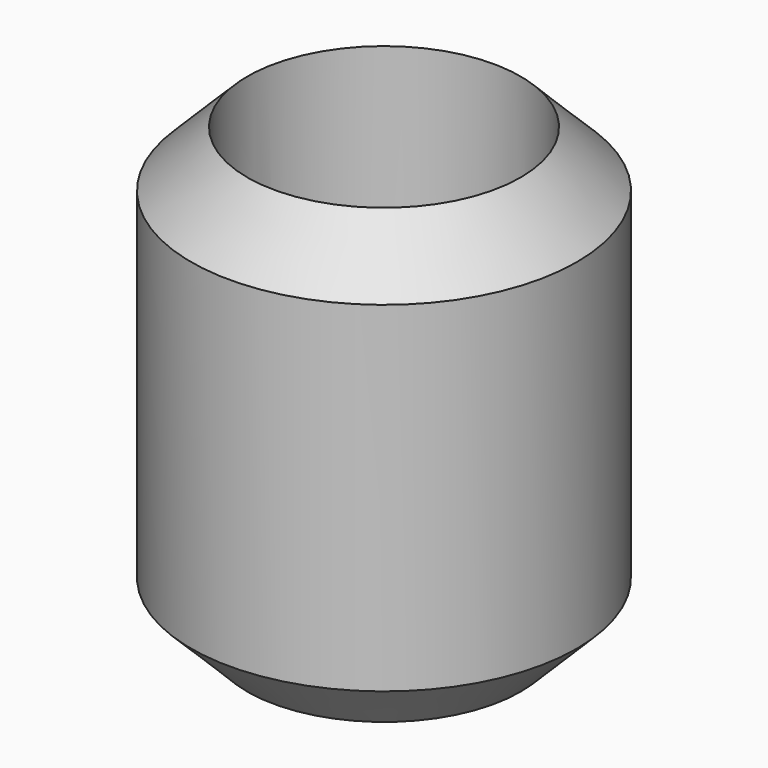
from build123d import *

# Parameters (mm, degrees)
F0_R     = 15.875
F0_R_2   = 11.25
F1_DEPTH = 38
F2_R     = 4
F4_DEPTH = 15.876


# Not quite as in the source:
# - a fillet or chamfer that OpenCascade refuses, or shapes differently, is made with other operations: its cross-section is extruded or revolved along the edge and cut away or added


with BuildPart() as f1:
    # F0 (on Top) → F1 (new body)
    with BuildSketch(Plane.XY):
        Circle(F0_R)
        Circle(F0_R_2, mode=Mode.SUBTRACT)
    extrude(amount=F1_DEPTH)

    # F3: chamfer of 5 on 2 edges, made by hand

    # F3_s1 → F3_t2 (revolve, cut)
    with BuildSketch(Plane.XZ):
        Polygon((15.875, 33), (10.875, 38), (15.875, 38), align=None)
    revolve(axis=Axis((0, 0, 38), (0, 0, 1)), mode=Mode.SUBTRACT)

    # F3_s3 → F3_t4 (revolve, cut)
    with BuildSketch(Plane.XZ):
        Polygon((15.875, 5), (10.875, 0), (15.875, 0), align=None)
    revolve(axis=Axis((0, 0, 0), (0, 0, 1)), mode=Mode.SUBTRACT)

    # F2 (on Front) → F4 (cut, through all)
    with BuildSketch(Plane.XZ):
        with Locations((7, 19)):
            Circle(F2_R)
        with Locations((-7, 19)):
            Circle(F2_R)
    extrude(amount=-F4_DEPTH, mode=Mode.SUBTRACT)


solid = f1.part
